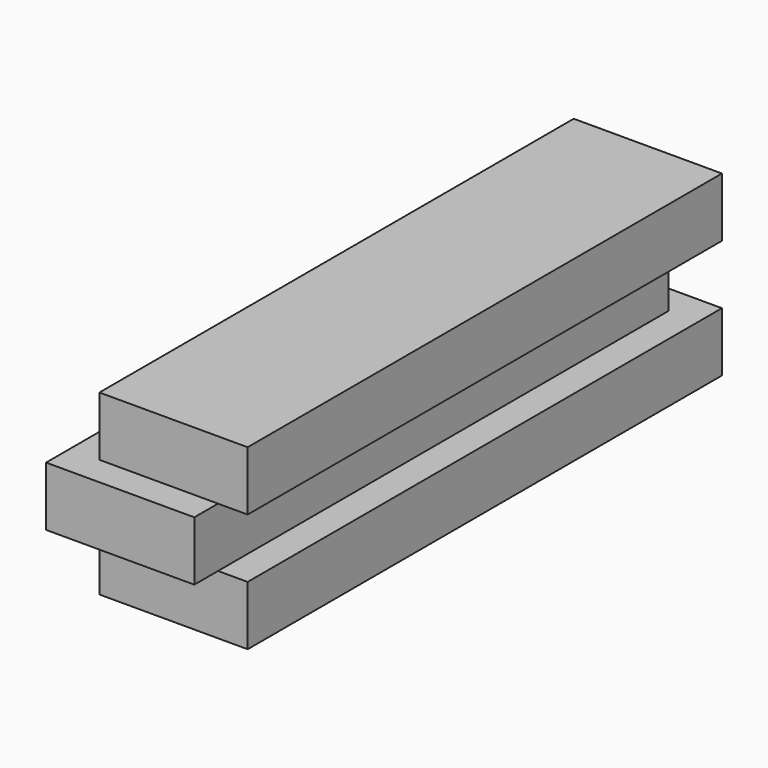
from build123d import *

# Parameters (mm, degrees)
F2_W     = 7.9375
F2_H     = 31.75
F3_DEPTH = 3.175
F4_W     = 7.9375
F4_H     = 31.75
F5_DEPTH = 3.175
F6_W     = 7.9375
F6_H     = 31.75
F7_DEPTH = 3.175


# Not quite as in the source:
# - a variable given as a bare number and used for a length is read in inches; the dataset says mm whatever the document's units were


with BuildPart() as f3:
    # F2 (on Top) → F3 (new body)
    with BuildSketch(Plane.XY):
        with Locations((3.96875, 15.875)):
            Rectangle(F2_W, F2_H)
    extrude(amount=F3_DEPTH)

    # F4 (on face) → F5 (join)
    with BuildSketch(Plane.XY.offset(3.175)):
        with Locations((2.38125, 14.2875)):
            Rectangle(F4_W, F4_H)
    extrude(amount=F5_DEPTH)

    # F6 (on face) → F7 (join)
    with BuildSketch(Plane.XY.offset(6.35)):
        with Locations((3.96875, 15.875)):
            Rectangle(F6_W, F6_H)
    extrude(amount=F7_DEPTH)


solid = f3.part
